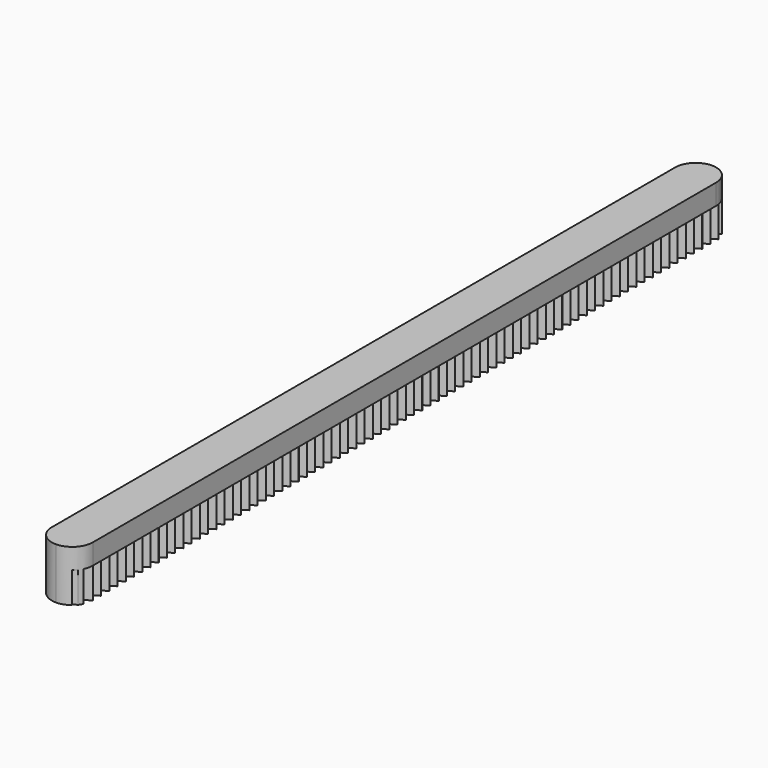
from build123d import *

# Parameters (mm, degrees)
F0_W     = 20
F0_H     = 400
F1_DEPTH = 25
F3_R     = 9.99999
F4_DEPTH = 15


# Not quite as in the source:
# - a fillet or chamfer is up to 0.001 mm smaller than in the source, because OpenCascade refuses the exact size


with BuildPart() as f1:
    # F0 (on Top) → F1 (new body)
    with BuildSketch(Plane.XY):
        Rectangle(F0_W, F0_H)
    extrude(amount=F1_DEPTH)

    # F3 (radius 10 in the source; OpenCascade refuses exactly that, so slightly less here)
    f3_edges = [f1.edges().sort_by_distance(p)[0] for p in [
        (10, -200, 12.5),
        (-10, -200, 12.5),
        (10, 200, 12.5),
        (-10, 200, 12.5),
    ]]
    fillet(f3_edges, radius=F3_R)

    # F2 (on Top) → F4 (cut)
    with BuildSketch(Plane.XY):
        Polygon((10, -195), (5.6698729811, -197.5), (10, -200), align=None)
        Polygon((10, -189.98), (5.6698729811, -192.48), (10, -194.98), align=None)
        Polygon((10, -184.96), (5.6698729811, -187.46), (10, -189.96), align=None)
        Polygon((10, -179.94), (5.6698729811, -182.44), (10, -184.94), align=None)
        Polygon((10, -174.92), (5.6698729811, -177.42), (10, -179.92), align=None)
        Polygon((10, -169.9), (5.6698729811, -172.4), (10, -174.9), align=None)
        Polygon((10, -164.88), (5.6698729811, -167.38), (10, -169.88), align=None)
        Polygon((10, -159.86), (5.6698729811, -162.36), (10, -164.86), align=None)
        Polygon((10, -154.84), (5.6698729811, -157.34), (10, -159.84), align=None)
        Polygon((10, -149.82), (5.6698729811, -152.32), (10, -154.82), align=None)
        Polygon((10, -144.8), (5.6698729811, -147.3), (10, -149.8), align=None)
        Polygon((10, -139.78), (5.6698729811, -142.28), (10, -144.78), align=None)
        Polygon((10, -134.76), (5.6698729811, -137.26), (10, -139.76), align=None)
        Polygon((10, -129.74), (5.6698729811, -132.24), (10, -134.74), align=None)
        Polygon((10, -124.72), (5.6698729811, -127.22), (10, -129.72), align=None)
        Polygon((10, -119.7), (5.6698729811, -122.2), (10, -124.7), align=None)
        Polygon((10, -114.68), (5.6698729811, -117.18), (10, -119.68), align=None)
        Polygon((10, -109.66), (5.6698729811, -112.16), (10, -114.66), align=None)
        Polygon((10, -104.64), (5.6698729811, -107.14), (10, -109.64), align=None)
        Polygon((10, -99.62), (5.6698729811, -102.12), (10, -104.62), align=None)
        Polygon((10, -94.6), (5.6698729811, -97.1), (10, -99.6), align=None)
        Polygon((10, -89.58), (5.6698729811, -92.08), (10, -94.58), align=None)
        Polygon((10, -84.56), (5.6698729811, -87.06), (10, -89.56), align=None)
        Polygon((10, -79.54), (5.6698729811, -82.04), (10, -84.54), align=None)
        Polygon((10, -74.52), (5.6698729811, -77.02), (10, -79.52), align=None)
        Polygon((10, -69.5), (5.6698729811, -72), (10, -74.5), align=None)
        Polygon((10, -64.48), (5.6698729811, -66.98), (10, -69.48), align=None)
        Polygon((10, -59.46), (5.6698729811, -61.96), (10, -64.46), align=None)
        Polygon((10, -54.44), (5.6698729811, -56.94), (10, -59.44), align=None)
        Polygon((10, -49.42), (5.6698729811, -51.92), (10, -54.42), align=None)
        Polygon((10, -44.4), (5.6698729811, -46.9), (10, -49.4), align=None)
        Polygon((10, -39.38), (5.6698729811, -41.88), (10, -44.38), align=None)
        Polygon((10, -34.36), (5.6698729811, -36.86), (10, -39.36), align=None)
        Polygon((10, -29.34), (5.6698729811, -31.84), (10, -34.34), align=None)
        Polygon((10, -24.32), (5.6698729811, -26.82), (10, -29.32), align=None)
        Polygon((10, -19.3), (5.6698729811, -21.8), (10, -24.3), align=None)
        Polygon((10, -14.28), (5.6698729811, -16.78), (10, -19.28), align=None)
        Polygon((10, -9.26), (5.6698729811, -11.76), (10, -14.26), align=None)
        Polygon((10, -4.24), (5.6698729811, -6.74), (10, -9.24), align=None)
        Polygon((10, 0.78), (5.6698729811, -1.72), (10, -4.22), align=None)
        Polygon((10, 5.8), (5.6698729811, 3.3), (10, 0.8), align=None)
        Polygon((10, 10.82), (5.6698729811, 8.32), (10, 5.82), align=None)
        Polygon((10, 15.84), (5.6698729811, 13.34), (10, 10.84), align=None)
        Polygon((10, 20.86), (5.6698729811, 18.36), (10, 15.86), align=None)
        Polygon((10, 25.88), (5.6698729811, 23.38), (10, 20.88), align=None)
        Polygon((10, 30.9), (5.6698729811, 28.4), (10, 25.9), align=None)
        Polygon((10, 35.92), (5.6698729811, 33.42), (10, 30.92), align=None)
        Polygon((10, 40.94), (5.6698729811, 38.44), (10, 35.94), align=None)
        Polygon((10, 45.96), (5.6698729811, 43.46), (10, 40.96), align=None)
        Polygon((10, 50.98), (5.6698729811, 48.48), (10, 45.98), align=None)
        Polygon((10, 56), (5.6698729811, 53.5), (10, 51), align=None)
        Polygon((10, 61.02), (5.6698729811, 58.52), (10, 56.02), align=None)
        Polygon((10, 66.04), (5.6698729811, 63.54), (10, 61.04), align=None)
        Polygon((10, 71.06), (5.6698729811, 68.56), (10, 66.06), align=None)
        Polygon((10, 76.08), (5.6698729811, 73.58), (10, 71.08), align=None)
        Polygon((10, 81.1), (5.6698729811, 78.6), (10, 76.1), align=None)
        Polygon((10, 86.12), (5.6698729811, 83.62), (10, 81.12), align=None)
        Polygon((10, 91.14), (5.6698729811, 88.64), (10, 86.14), align=None)
        Polygon((10, 96.16), (5.6698729811, 93.66), (10, 91.16), align=None)
        Polygon((10, 101.18), (5.6698729811, 98.68), (10, 96.18), align=None)
        Polygon((10, 106.2), (5.6698729811, 103.7), (10, 101.2), align=None)
        Polygon((10, 111.22), (5.6698729811, 108.72), (10, 106.22), align=None)
        Polygon((10, 116.24), (5.6698729811, 113.74), (10, 111.24), align=None)
        Polygon((10, 121.26), (5.6698729811, 118.76), (10, 116.26), align=None)
        Polygon((10, 126.28), (5.6698729811, 123.78), (10, 121.28), align=None)
        Polygon((10, 131.3), (5.6698729811, 128.8), (10, 126.3), align=None)
        Polygon((10, 136.32), (5.6698729811, 133.82), (10, 131.32), align=None)
        Polygon((10, 141.34), (5.6698729811, 138.84), (10, 136.34), align=None)
        Polygon((10, 146.36), (5.6698729811, 143.86), (10, 141.36), align=None)
        Polygon((10, 151.38), (5.6698729811, 148.88), (10, 146.38), align=None)
        Polygon((10, 156.4), (5.6698729811, 153.9), (10, 151.4), align=None)
        Polygon((10, 161.42), (5.6698729811, 158.92), (10, 156.42), align=None)
        Polygon((10, 166.44), (5.6698729811, 163.94), (10, 161.44), align=None)
        Polygon((10, 171.46), (5.6698729811, 168.96), (10, 166.46), align=None)
        Polygon((10, 176.48), (5.6698729811, 173.98), (10, 171.48), align=None)
        Polygon((10, 181.5), (5.6698729811, 179), (10, 176.5), align=None)
        Polygon((10, 186.52), (5.6698729811, 184.02), (10, 181.52), align=None)
        Polygon((10, 191.54), (5.6698729811, 189.04), (10, 186.54), align=None)
        Polygon((10, 196.56), (5.6698729811, 194.06), (10, 191.56), align=None)
        Polygon((10, 201.58), (5.6698729811, 199.08), (10, 196.58), align=None)
        Polygon((10, 206.6), (5.6698729811, 204.1), (10, 201.6), align=None)
        Polygon((10, 211.62), (5.6698729811, 209.12), (10, 206.62), align=None)
        Polygon((10, 216.64), (5.6698729811, 214.14), (10, 211.64), align=None)
        Polygon((10, 221.66), (5.6698729811, 219.16), (10, 216.66), align=None)
        Polygon((10, 226.68), (5.6698729811, 224.18), (10, 221.68), align=None)
        Polygon((10, 231.7), (5.6698729811, 229.2), (10, 226.7), align=None)
        Polygon((10, 236.72), (5.6698729811, 234.22), (10, 231.72), align=None)
        Polygon((10, 241.74), (5.6698729811, 239.24), (10, 236.74), align=None)
        Polygon((10, 246.76), (5.6698729811, 244.26), (10, 241.76), align=None)
        Polygon((10, 251.78), (5.6698729811, 249.28), (10, 246.78), align=None)
        Polygon((10, 256.8), (5.6698729811, 254.3), (10, 251.8), align=None)
        Polygon((10, 261.82), (5.6698729811, 259.32), (10, 256.82), align=None)
        Polygon((10, 266.84), (5.6698729811, 264.34), (10, 261.84), align=None)
        Polygon((10, 271.86), (5.6698729811, 269.36), (10, 266.86), align=None)
        Polygon((10, 276.88), (5.6698729811, 274.38), (10, 271.88), align=None)
        Polygon((10, 281.9), (5.6698729811, 279.4), (10, 276.9), align=None)
        Polygon((10, 286.92), (5.6698729811, 284.42), (10, 281.92), align=None)
        Polygon((10, 291.94), (5.6698729811, 289.44), (10, 286.94), align=None)
        Polygon((10, 296.96), (5.6698729811, 294.46), (10, 291.96), align=None)
        Polygon((10, 301.98), (5.6698729811, 299.48), (10, 296.98), align=None)
    extrude(amount=F4_DEPTH, mode=Mode.SUBTRACT)


solid = f1.part
